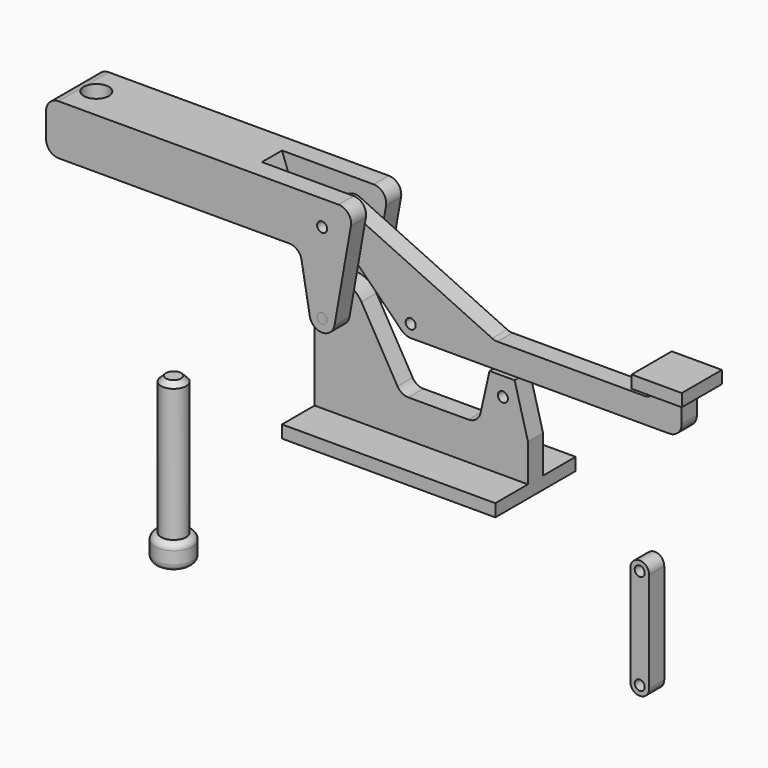
from build123d import *

# Parameters (mm, degrees)
F6_SIZE2  = 1.27
F6_SIZE   = 1.27
F3_R      = 1.27
F7_DEPTH  = 2.3876
F2_W      = 53.975
F2_H      = 3.175
F8_DEPTH  = 12.7
F2_R      = 1.27
F9_DEPTH  = 2.3876
F0_R      = 1.27
F10_DEPTH = 2.3876
F11_DEPTH = 6.35
F1_R      = 1.27
F12_DEPTH = 7.9375
F13_W     = 12.7
F13_H     = 6.35
F14_DEPTH = 53.595
F16_DEPTH = 6.35
F18_D     = 6.35
F19_DEPTH = 7.9375


# Not quite as in the source:
# - ends of sketch curves that miss each other by under 0.0002 mm in the source are joined


with BuildPart() as f5:
    # F4 (on Front) → F5 (revolve)
    with BuildSketch(Plane.XZ):
        with BuildLine():
            Line((-58.7122046471, -67.5823132604), (-58.7122046471, -32.6573132604))
            Line((-58.7122046471, -32.6573132604), (-61.8872046471, -32.6573132604))
            Line((-61.8872046471, -32.6573132604), (-61.8872046471, -73.9323132604))
            Line((-61.8872046471, -73.9323132604), (-58.7249046471, -73.9323132604))
            ThreePointArc((-58.7249046471, -73.9323132604), (-57.5933923758, -73.4636255317), (-57.1247046471, -72.3321132604))
            Line((-57.1247046471, -72.3321132604), (-57.1247046471, -69.1825132604))
            ThreePointArc((-57.1247046471, -69.1825132604), (-57.5889112624, -68.0554999198), (-58.7122046471, -67.5823132604))
        make_face()
    revolve(axis=Axis((-61.8872046471, 0, -53.2948132604), (0, 0, -1)))

    # F6
    f6_edges = [f5.edges().sort_by_distance(p)[0] for p in [
        (-65.062205, 0, -32.657313),
    ]]
    chamfer(f6_edges, length=F6_SIZE, length2=F6_SIZE2)


with BuildPart() as f7:
    # F3 (on Front) → F7 (new body, symmetric)
    with BuildSketch(Plane.XZ):
        with BuildLine():
            Line((60.335984434, -61.6455189884), (60.335984434, -36.2455189884))
            ThreePointArc((60.335984434, -36.2455189884), (57.948384434, -33.8579189884), (55.560784434, -36.2455189884))
            Line((55.560784434, -36.2455189884), (55.560784434, -61.6455189884))
            ThreePointArc((55.560784434, -61.6455189884), (57.948384434, -64.0331189884), (60.335984434, -61.6455189884))
        make_face()
        with Locations((57.948384434, -61.6455189884)):
            Circle(F3_R, mode=Mode.SUBTRACT)
        with Locations((57.948384434, -36.2455189884)):
            Circle(F3_R, mode=Mode.SUBTRACT)
    extrude(amount=F7_DEPTH, both=True)


with BuildPart() as f8:
    # F2 (on Front) → F8 (new body, symmetric)
    with BuildSketch(Plane.XZ):
        with Locations((2.6769877579, -27.6959877579)):
            Rectangle(F2_W, F2_H)
    extrude(amount=F8_DEPTH, both=True)

    # F2 (on Front) → F9 (join, symmetric)
    with BuildSketch(Plane.XZ):
        with BuildLine():
            Line((-3.3324771468, -14.9959877579), (-12.4612509281, 0.8155122421))
            ThreePointArc((-12.4612509281, 0.8155122421), (-19.6040131785, 3.7741412391), (-24.3105122421, -2.3594877579))
            Line((-24.3105122421, -2.3594877579), (-24.3105122421, -26.1084877579))
            Line((-24.3105122421, -26.1084877579), (29.6644877579, -26.1084877579))
            Line((29.6644877579, -26.1084877579), (29.6644877579, -16.5834877579))
            Line((29.6644877579, -16.5834877579), (26.2955625614, -4.0104877579))
            Line((26.2955625614, -4.0104877579), (19.9455625614, -4.0104877579))
            Line((19.9455625614, -4.0104877579), (17.677843549, -14.1044398719))
            ThreePointArc((17.677843549, -14.1044398719), (16.5638645169, -15.8874263374), (14.5800579439, -16.5834877579))
            Line((14.5800579439, -16.5834877579), (-0.5828464898, -16.5834877579))
            ThreePointArc((-0.5828464898, -16.5834877579), (-2.1703464898, -16.1581184149), (-3.3324771468, -14.9959877579))
        make_face()
        with Locations((-17.9605122421, -2.3594877579)):
            Circle(F2_R, mode=Mode.SUBTRACT)
        with Locations((23.3144877579, -8.7094877579)):
            Circle(F2_R, mode=Mode.SUBTRACT)
    extrude(amount=F9_DEPTH, both=True)


with BuildPart() as f10:
    # F0 (on Front) → F10 (new body, symmetric)
    with BuildSketch(Plane.XZ):
        with BuildLine():
            ThreePointArc((-2.2450640303, -2.2450640303), (-1.2150198978, -2.9333175157), (0, -3.175))
            Line((0, -3.175), (59.055, -3.175))
            Line((59.055, -3.175), (65.405, -3.175))
            ThreePointArc((65.405, -3.175), (67.6500640303, -2.2450640303), (68.58, 0))
            Line((68.58, 0), (68.58, 6.35))
            Line((68.58, 6.35), (62.23, 6.35))
            ThreePointArc((62.23, 6.35), (61.3000640303, 4.1049359697), (59.055, 3.175))
            Line((59.055, 3.175), (21.9636916648, 3.175))
            ThreePointArc((21.9636916648, 3.175), (21.2764958906, 3.2502601774), (20.6218786838, 3.4724727762))
            Line((20.6218786838, 3.4724727762), (-16.6186992611, 20.838039466))
            ThreePointArc((-16.6186992611, 20.838039466), (-20.5613199828, 19.7816174276), (-20.2055762724, 15.7154482119))
            Line((-20.2055762724, 15.7154482119), (-2.2450640303, -2.2450640303))
        make_face()
        Circle(F0_R, mode=Mode.SUBTRACT)
        with Locations((-17.9605122421, 17.9605122421)):
            Circle(F0_R, mode=Mode.SUBTRACT)
    extrude(amount=F10_DEPTH, both=True)

    # F0 (on Front) → F11 (join, symmetric)
    with BuildSketch(Plane.XZ):
        Polygon((62.23, 6.35), (68.58, 6.35), (71.755, 6.35), (71.755, 9.525), (59.055, 9.525), (59.055, 6.35), align=None)
    extrude(amount=F11_DEPTH, both=True)


with BuildPart() as f12:
    # F1 (on Front) → F12 (new body, symmetric)
    with BuildSketch(Plane.XZ):
        with BuildLine():
            ThreePointArc((-21.087276858, -2.910820722), (-18.2372317254, 0.8034304086), (-14.7855122421, -2.3594877579))
            ThreePointArc((-14.7855122421, -2.3594877579), (-14.7975940757, -2.6362072411), (-14.8337476263, -2.910820722))
            Line((-14.8337476263, -2.910820722), (-10.6909452146, 20.584179278))
            ThreePointArc((-10.6909452146, 20.584179278), (-11.3855187235, 23.1763629029), (-13.8177098304, 24.3105122421))
            Line((-13.8177098304, 24.3105122421), (-84.6355122421, 24.3105122421))
            ThreePointArc((-84.6355122421, 24.3105122421), (-86.8805762724, 23.3805762724), (-87.8105122421, 21.1355122421))
            Line((-87.8105122421, 21.1355122421), (-87.8105122421, 14.7855122421))
            ThreePointArc((-87.8105122421, 14.7855122421), (-86.8805762724, 12.5404482119), (-84.6355122421, 11.6105122421))
            Line((-84.6355122421, 11.6105122421), (-26.3119209844, 11.6105122421))
            ThreePointArc((-26.3119209844, 11.6105122421), (-24.2710703236, 10.867703349), (-23.1851563685, 8.9868452062))
            Line((-23.1851563685, 8.9868452062), (-21.087276858, -2.910820722))
        make_face()
        with Locations((-17.9605122421, 17.9605122421)):
            Circle(F1_R, mode=Mode.SUBTRACT)
        with BuildLine():
            ThreePointArc((-14.8337476263, -2.910820722), (-14.7975940757, -2.6362072411), (-14.7855122421, -2.3594877579))
            ThreePointArc((-14.7855122421, -2.3594877579), (-18.2372317254, 0.8034304086), (-21.087276858, -2.910820722))
            ThreePointArc((-21.087276858, -2.910820722), (-17.9605122421, -5.5344877579), (-14.8337476263, -2.910820722))
        make_face()
        with Locations((-17.9605122421, -2.3594877579)):
            Circle(F1_R, mode=Mode.SUBTRACT)
    extrude(amount=F12_DEPTH, both=True)

    # F13 (on face) → F14 (cut, through all)
    with BuildSketch(Plane(origin=(0, 0, -29.2834877579), x_dir=(1, 0, 0), z_dir=(0, 0, -1))):
        with Locations((-30.6605122421, 0)):
            Rectangle(F13_W, F13_H)
        Polygon((29.6644877579, -2.3876), (29.6644877579, 2.3876), (29.6644877579, 3.175), (-24.3105122421, 3.175), (-24.3105122421, -3.175), (29.6644877579, -3.175), align=None)
    extrude(amount=-F14_DEPTH, mode=Mode.SUBTRACT)

    # F15 (on face) → F16 (join, through all)
    with BuildSketch(Plane.XZ.offset(-3.175)):
        Polygon((-32.388090267, 11.6105122421), (-37.0105122421, 24.3105122421), (-37.0105122421, 11.6105122421), align=None)
    extrude(amount=F16_DEPTH)

    # F18 (through all)
    with Locations(Plane.XY.offset(24.3105122421)):
        with Locations((-81.4605122421, 0)):
            Hole(F18_D / 2)


with BuildPart() as f19:
    # F1 (on Front) → F19 (new body, symmetric)
    with BuildSketch(Plane.XZ):
        with Locations((-17.9605122421, -2.3594877579)):
            Circle(F1_R)
    extrude(amount=F19_DEPTH, both=True)


solid = Compound([f5.part, f7.part, f8.part, f10.part, f12.part, f19.part])
